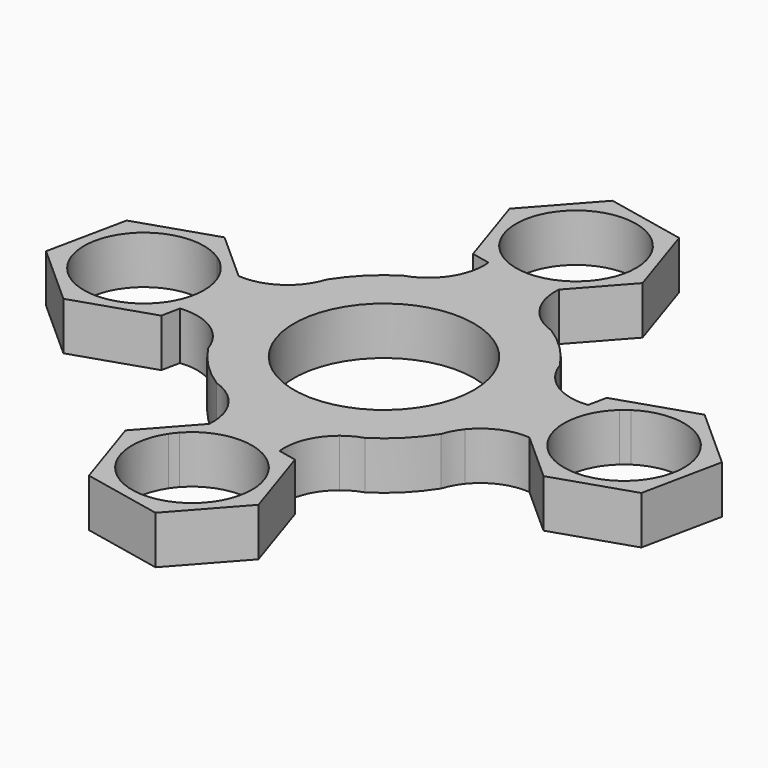
from build123d import *

# Parameters (mm, degrees)
F0_R     = 7.5
F1_DEPTH = 4


with BuildPart() as f1:
    # F0 (on Top) → F1 (new body)
    with BuildSketch(Plane.XY):
        with BuildLine():
            ThreePointArc((10.5023390129, 4.6851761182), (10.0305689983, 5.3963431452), (9.6971069971, 6.1819184634))
            ThreePointArc((9.6971069971, 6.1819184634), (8.1317279836, 8.1317279836), (6.1819184634, 9.6971069971))
            ThreePointArc((6.1819184634, 9.6971069971), (5.3963431452, 10.0305689983), (4.6851761182, 10.5023390129))
            ThreePointArc((4.6851761182, 10.5023390129), (0, 11.5), (-4.6851761182, 10.5023390129))
            ThreePointArc((-4.6851761182, 10.5023390129), (-5.3963431452, 10.0305689983), (-6.1819184634, 9.6971069971))
            ThreePointArc((-6.1819184634, 9.6971069971), (-8.1317279836, 8.1317279836), (-9.6971069971, 6.1819184634))
            ThreePointArc((-9.6971069971, 6.1819184634), (-10.0305689983, 5.3963431452), (-10.5023390129, 4.6851761182))
            ThreePointArc((-10.5023390129, 4.6851761182), (-11.5, 0), (-10.5023390129, -4.6851761182))
            ThreePointArc((-10.5023390129, -4.6851761182), (-10.0305689983, -5.3963431452), (-9.6971069971, -6.1819184634))
            ThreePointArc((-9.6971069971, -6.1819184634), (-8.1317279836, -8.1317279836), (-6.1819184634, -9.6971069971))
            ThreePointArc((-6.1819184634, -9.6971069971), (-5.3963431452, -10.0305689983), (-4.6851761182, -10.5023390129))
            ThreePointArc((-4.6851761182, -10.5023390129), (0, -11.5), (4.6851761182, -10.5023390129))
            ThreePointArc((4.6851761182, -10.5023390129), (5.3963431452, -10.0305689983), (6.1819184634, -9.6971069971))
            ThreePointArc((6.1819184634, -9.6971069971), (8.1317279836, -8.1317279836), (9.6971069971, -6.1819184634))
            ThreePointArc((9.6971069971, -6.1819184634), (10.0305689983, -5.3963431452), (10.5023390129, -4.6851761182))
            ThreePointArc((10.5023390129, -4.6851761182), (11.2478197587, -2.3951097419), (11.5, 0))
            ThreePointArc((11.5, 0), (11.2478197587, 2.3951097419), (10.5023390129, 4.6851761182))
        make_face()
        Circle(F0_R, mode=Mode.SUBTRACT)
        with BuildLine():
            ThreePointArc((14.6103055623, 2.982595382), (12.338941223, 3.3093913031), (10.5023390129, 4.6851761182))
            ThreePointArc((10.5023390129, 4.6851761182), (11.2478197587, 2.3951097419), (11.5, 0))
            ThreePointArc((11.5, 0), (11.2478197587, -2.3951097419), (10.5023390129, -4.6851761182))
            ThreePointArc((10.5023390129, -4.6851761182), (12.2847026286, -3.3322754018), (14.4930952607, -2.9714951504))
            ThreePointArc((14.4930952607, -2.9714951504), (15.6148030882, -3.2054073782), (16.6449174053, -3.7072119959))
            ThreePointArc((16.6449174053, -3.7072119959), (15, 0), (16.6449174053, 3.7072119959))
            ThreePointArc((16.6449174053, 3.7072119959), (15.6703838257, 3.2248055408), (14.6103055623, 2.982595382))
        make_face()
        with BuildLine():
            ThreePointArc((-4.6851761182, 10.5023390129), (0, 11.5), (4.6851761182, 10.5023390129))
            ThreePointArc((4.6851761182, 10.5023390129), (3.3322754018, 12.2847026286), (2.9714951504, 14.4930952607))
            ThreePointArc((2.9714951504, 14.4930952607), (3.2054073782, 15.6148030882), (3.7072119959, 16.6449174053))
            ThreePointArc((3.7072119959, 16.6449174053), (0, 15), (-3.7072119959, 16.6449174053))
            ThreePointArc((-3.7072119959, 16.6449174053), (-3.2248055408, 15.6703838257), (-2.982595382, 14.6103055623))
            ThreePointArc((-2.982595382, 14.6103055623), (-3.3093913031, 12.338941223), (-4.6851761182, 10.5023390129))
        make_face()
        with BuildLine():
            Line((14.9337128596, 4.5302571293), (14.6103055623, 2.982595382))
            ThreePointArc((14.6103055623, 2.982595382), (15.6703838257, 3.2248055408), (16.6449174053, 3.7072119959))
            ThreePointArc((16.6449174053, 3.7072119959), (16.936960195, 3.9519346089), (17.2467904427, 4.17370784))
            ThreePointArc((17.2467904427, 4.17370784), (22.3700160562, 4.4026155741), (25, 0))
            ThreePointArc((25, 0), (22.3700160562, -4.4026155741), (17.2467904427, -4.17370784))
            ThreePointArc((17.2467904427, -4.17370784), (16.936960195, -3.9519346089), (16.6449174053, -3.7072119959))
            ThreePointArc((16.6449174053, -3.7072119959), (15.6148030882, -3.2054073782), (14.4930952607, -2.9714951504))
            Line((14.4930952607, -2.9714951504), (18.6098258106, -6.6526619311))
            Line((18.6098258106, -6.6526619311), (25.0662871404, -4.5302571293))
            Line((25.0662871404, -4.5302571293), (26.4564613299, 2.1224048018))
            Line((26.4564613299, 2.1224048018), (21.3901741894, 6.6526619311))
            Line((21.3901741894, 6.6526619311), (14.9337128596, 4.5302571293))
        make_face()
        with BuildLine():
            ThreePointArc((3.7072119959, 16.6449174053), (3.2054073782, 15.6148030882), (2.9714951504, 14.4930952607))
            Line((2.9714951504, 14.4930952607), (6.6526619311, 18.6098258106))
            Line((6.6526619311, 18.6098258106), (4.5302571293, 25.0662871404))
            Line((4.5302571293, 25.0662871404), (-2.1224048018, 26.4564613299))
            Line((-2.1224048018, 26.4564613299), (-6.6526619311, 21.3901741894))
            Line((-6.6526619311, 21.3901741894), (-4.5302571293, 14.9337128596))
            Line((-4.5302571293, 14.9337128596), (-2.982595382, 14.6103055623))
            ThreePointArc((-2.982595382, 14.6103055623), (-3.2248055408, 15.6703838257), (-3.7072119959, 16.6449174053))
            ThreePointArc((-3.7072119959, 16.6449174053), (-3.9519346089, 16.936960195), (-4.17370784, 17.2467904427))
            ThreePointArc((-4.17370784, 17.2467904427), (-1.4372649025, 24.7889737523), (5, 20))
            ThreePointArc((5, 20), (4.7889737523, 18.5627350975), (4.17370784, 17.2467904427))
            ThreePointArc((4.17370784, 17.2467904427), (3.9519346089, 16.936960195), (3.7072119959, 16.6449174053))
        make_face()
        with BuildLine():
            ThreePointArc((-10.5023390129, -4.6851761182), (-11.5, 0), (-10.5023390129, 4.6851761182))
            ThreePointArc((-10.5023390129, 4.6851761182), (-12.2847026286, 3.3322754018), (-14.4930952607, 2.9714951504))
            ThreePointArc((-14.4930952607, 2.9714951504), (-15.6148030882, 3.2054073782), (-16.6449174053, 3.7072119959))
            ThreePointArc((-16.6449174053, 3.7072119959), (-15.4296929549, 2.0278790677), (-15, 0))
            ThreePointArc((-15, 0), (-15.4296929549, -2.0278790677), (-16.6449174053, -3.7072119959))
            ThreePointArc((-16.6449174053, -3.7072119959), (-15.6703838257, -3.2248055408), (-14.6103055623, -2.982595382))
            ThreePointArc((-14.6103055623, -2.982595382), (-12.338941223, -3.3093913031), (-10.5023390129, -4.6851761182))
        make_face()
        with BuildLine():
            ThreePointArc((2.982595382, -14.6103055623), (3.3093913031, -12.338941223), (4.6851761182, -10.5023390129))
            ThreePointArc((4.6851761182, -10.5023390129), (0, -11.5), (-4.6851761182, -10.5023390129))
            ThreePointArc((-4.6851761182, -10.5023390129), (-3.3322754018, -12.2847026286), (-2.9714951504, -14.4930952607))
            ThreePointArc((-2.9714951504, -14.4930952607), (-3.2054073782, -15.6148030882), (-3.7072119959, -16.6449174053))
            ThreePointArc((-3.7072119959, -16.6449174053), (0, -15), (3.7072119959, -16.6449174053))
            ThreePointArc((3.7072119959, -16.6449174053), (3.2248055408, -15.6703838257), (2.982595382, -14.6103055623))
        make_face()
        with BuildLine():
            ThreePointArc((-16.6449174053, 3.7072119959), (-15.6148030882, 3.2054073782), (-14.4930952607, 2.9714951504))
            Line((-14.4930952607, 2.9714951504), (-18.6098258106, 6.6526619311))
            Line((-18.6098258106, 6.6526619311), (-25.0662871404, 4.5302571293))
            Line((-25.0662871404, 4.5302571293), (-26.4564613299, -2.1224048018))
            Line((-26.4564613299, -2.1224048018), (-21.3901741894, -6.6526619311))
            Line((-21.3901741894, -6.6526619311), (-14.9337128596, -4.5302571293))
            Line((-14.9337128596, -4.5302571293), (-14.6103055623, -2.982595382))
            ThreePointArc((-14.6103055623, -2.982595382), (-15.6703838257, -3.2248055408), (-16.6449174053, -3.7072119959))
            ThreePointArc((-16.6449174053, -3.7072119959), (-16.936960195, -3.9519346089), (-17.2467904427, -4.17370784))
            ThreePointArc((-17.2467904427, -4.17370784), (-25, 0), (-17.2467904427, 4.17370784))
            ThreePointArc((-17.2467904427, 4.17370784), (-16.936960195, 3.9519346089), (-16.6449174053, 3.7072119959))
        make_face()
        with BuildLine():
            Line((4.5302571293, -14.9337128596), (2.982595382, -14.6103055623))
            ThreePointArc((2.982595382, -14.6103055623), (3.2248055408, -15.6703838257), (3.7072119959, -16.6449174053))
            ThreePointArc((3.7072119959, -16.6449174053), (3.9519346089, -16.936960195), (4.17370784, -17.2467904427))
            ThreePointArc((4.17370784, -17.2467904427), (4.7889737523, -18.5627350975), (5, -20))
            ThreePointArc((5, -20), (-1.4372649025, -24.7889737523), (-4.17370784, -17.2467904427))
            ThreePointArc((-4.17370784, -17.2467904427), (-3.9519346089, -16.936960195), (-3.7072119959, -16.6449174053))
            ThreePointArc((-3.7072119959, -16.6449174053), (-3.2054073782, -15.6148030882), (-2.9714951504, -14.4930952607))
            Line((-2.9714951504, -14.4930952607), (-6.6526619311, -18.6098258106))
            Line((-6.6526619311, -18.6098258106), (-4.5302571293, -25.0662871404))
            Line((-4.5302571293, -25.0662871404), (2.1224048018, -26.4564613299))
            Line((2.1224048018, -26.4564613299), (6.6526619311, -21.3901741894))
            Line((6.6526619311, -21.3901741894), (4.5302571293, -14.9337128596))
        make_face()
    extrude(amount=F1_DEPTH)


solid = f1.part
